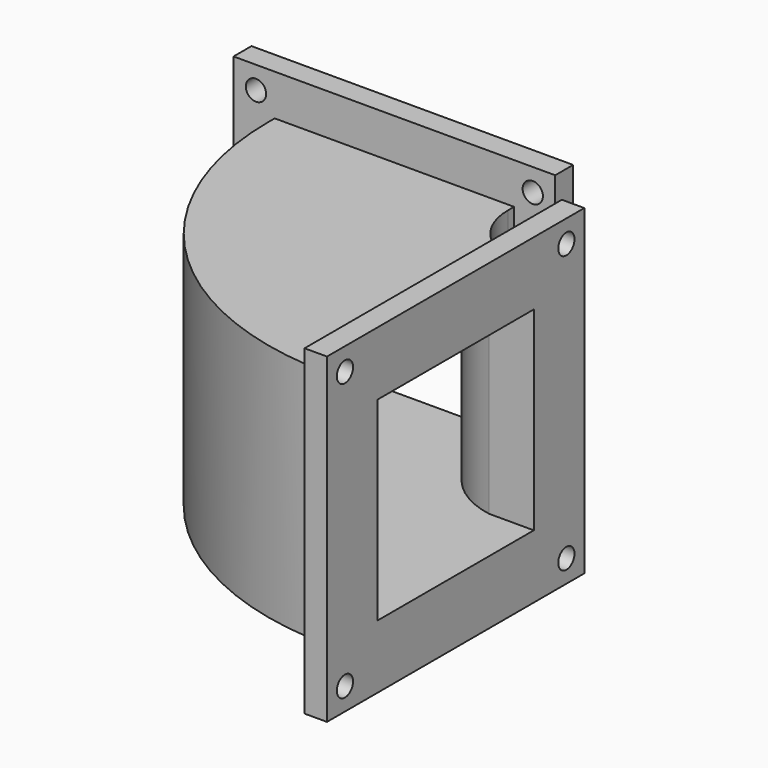
from build123d import *

# Parameters (mm, degrees)
F1_DEPTH = 50.8
F2_T     = -4.7625
F3_DEPTH = 4.7625
F4_W     = 68.2625
F4_H     = 68.2625
F4_R     = 2.15265
F4_W_2   = 50.8
F4_H_2   = 50.8
F4_W_3   = 41.4684797912
F4_H_3   = 41.275
F5_DEPTH = 4.7625
F6_W     = 68.2625
F6_H     = 68.2625
F6_R     = 2.15265
F6_W_2   = 41.275
F6_H_2   = 41.275
F7_DEPTH = 4.7625
F8_R     = 2.15265
F9_DEPTH = 74.6135


# Not quite as in the source:
# - a feature names something its author has since deleted; it is built from what else it names


with BuildPart() as f1:
    # F0 (on Top) → F1 (new body)
    with BuildSketch(Plane.XY):
        with BuildLine():
            ThreePointArc((13.49375, -13.49375), (3.9522278714, -9.5415221286), (0, 0))
            Line((0, 0), (0, 1.5875))
            Line((0, 1.5875), (-50.8, 1.5875))
            Line((-50.8, 1.5875), (-50.8, 0))
            ThreePointArc((-50.8, 0), (-31.9687966129, -45.4625466129), (13.49375, -64.29375))
            Line((13.49375, -64.29375), (15.08125, -64.29375))
            Line((15.08125, -64.29375), (15.08125, -13.49375))
            Line((15.08125, -13.49375), (13.49375, -13.49375))
        make_face()
    extrude(amount=F1_DEPTH)

    # F2
    f2_openings = [f1.faces().sort_by_distance(p)[0] for p in [
        (-25.4, 1.5875, 25.4),
    ]]
    offset(amount=F2_T, openings=f2_openings)

    # F3 (cut, through all): a face of the model
    f3_faces = [f1.faces().sort_by_distance(p)[0] for p in [
        (10.31875, -38.7122831446, 25.4),
    ]]
    extrude(f3_faces, amount=-F3_DEPTH, mode=Mode.SUBTRACT)

    # F4 (on face) → F5 (join)
    with BuildSketch(Plane.YZ.offset(15.08125)):
        with Locations((-38.7122831446, 25.4)):
            Rectangle(F4_W, F4_H)
        with Locations((-68.0810331446, -3.96875)):
            Circle(F4_R, mode=Mode.SUBTRACT)
        with Locations((-38.89375, 25.4)):
            Rectangle(F4_W_2, F4_H_2, mode=Mode.SUBTRACT)
        with Locations((-9.3435331446, -3.96875)):
            Circle(F4_R, mode=Mode.SUBTRACT)
        with Locations((-68.0810331446, 54.76875)):
            Circle(F4_R, mode=Mode.SUBTRACT)
        with Locations((-9.3435331446, 54.76875)):
            Circle(F4_R, mode=Mode.SUBTRACT)
        with Locations((-38.89375, 25.4)):
            Rectangle(F4_W_2, F4_H_2)
        with Locations((-38.7122831446, 25.4)):
            Rectangle(F4_W_3, F4_H_3, mode=Mode.SUBTRACT)
    extrude(amount=F5_DEPTH)

    # F6 (on face) → F7 (join)
    with BuildSketch(Plane(origin=(0, 1.5875, 0), x_dir=(-1, 0, 0), z_dir=(0, 1, 0))):
        with Locations((25.4, 25.4)):
            Rectangle(F6_W, F6_H)
        with Locations((-3.96875, -3.96875)):
            Circle(F6_R, mode=Mode.SUBTRACT)
        with Locations((54.76875, -3.96875)):
            Circle(F6_R, mode=Mode.SUBTRACT)
        with Locations((25.4, 25.4)):
            Rectangle(F6_W_2, F6_H_2, mode=Mode.SUBTRACT)
        with Locations((-3.96875, 54.76875)):
            Circle(F6_R, mode=Mode.SUBTRACT)
        with Locations((54.76875, 54.76875)):
            Circle(F6_R, mode=Mode.SUBTRACT)
    extrude(amount=F7_DEPTH)

    # F8 (on face) → F9 (cut, through all)
    with BuildSketch(Plane(origin=(15.08125, 0, 0), x_dir=(0, -1, 0), z_dir=(-1, 0, 0))):
        with BuildLine():
            ThreePointArc((68.0810331446, 59.53125), (64.7134370992, 51.4011539546), (72.8435331446, 54.76875))
            ThreePointArc((72.8435331446, 54.76875), (71.44862919, 58.1363460454), (68.0810331446, 59.53125))
        make_face()
        with Locations((68.0810331446, 54.76875)):
            Circle(F8_R, mode=Mode.SUBTRACT)
        with Locations((68.0810331446, 54.76875)):
            Circle(F8_R)
    extrude(amount=F9_DEPTH, mode=Mode.SUBTRACT)


solid = f1.part
